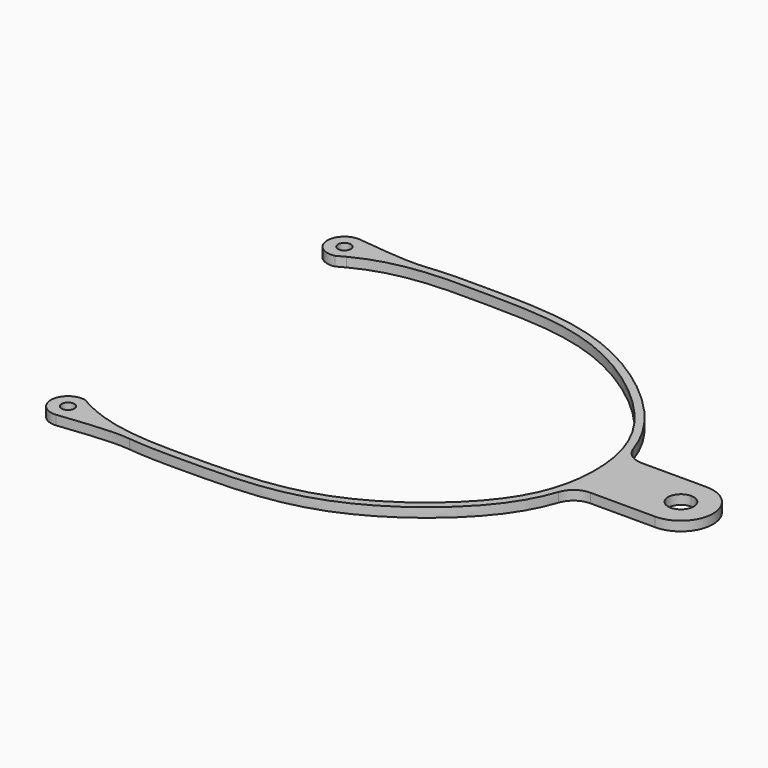
from build123d import *

# Parameters (mm, degrees)
F0_R     = 1.5
F1_DEPTH = 2.2
F2_R     = 5


# Not quite as in the source:
# - ends of sketch curves that miss each other by under 0.0002 mm in the source are joined
# - the dataset's text gives a spline's control points without its knots; the knots are read off the source's solid


with BuildPart() as f1:
    # F0 (on Top) → F1 (new body)
    with BuildSketch(Plane.XY):
        with BuildLine():
            add(Edge.make_bspline(
                [(-30.6111583346, -40.7008057443), (-31.233077321, -40.3790771173), (-31.8528544001, -40.0346551051), (-32.469697118, -39.6698600783)],
                knots=[0.6865550694, 0.6865550694, 0.6865550694, 0.6865550694, 0.698673585, 0.698673585, 0.698673585, 0.698673585], degree=3))
            ThreePointArc((-32.469697118, -39.6698600783), (-37.400344821, -43.2656468064), (-33.0455697059, -47.5407962381))
            add(Edge.make_bspline(
                [(-33.0455697059, -47.5407962381), (-28.2150059427, -47.0976245157), (-21.512714319, -46.0289871022), (-16.6916312134, -46.5655575872)],
                knots=[0, 0, 0, 0, 16.3829910165, 16.3829910165, 16.3829910165, 16.3829910165], degree=3))
            add(Edge.make_bspline(
                [(58.5705779891, -10.6833517733), (58.5045966245, -10.9937274451), (58.1139682264, -12.7078835649), (57.1321161632, -15.8212976201), (55.4627512009, -19.3062888881), (53.7559729129, -22.0784311932), (51.7889797877, -24.8398815578), (48.8824684734, -28.233839645), (44.8027944584, -32.1279022255), (40.2521320917, -35.7428568059), (35.3501612154, -38.9743729453), (31.0709874957, -41.2568133399), (27.5873440069, -42.7817363934), (24.0850094319, -44.0818391055), (19.7200729084, -45.2896051132), (14.5079732054, -46.2040279233), (9.333650913, -46.7087635295), (5.0560116744, -46.8940848045), (1.6559105615, -46.9634870038), (-0.8844247603, -46.9908203291), (-3.4095063019, -47.0107743311), (-5.9465324466, -47.0289364293), (-8.4959599535, -47.0211705077), (-11.9085350935, -46.9496883405), (-14.6448180595, -46.7853276586), (-16.5270909923, -46.5838707043), (-16.6916312134, -46.5655575872)],
                knots=[0.0555924477, 0.0555924477, 0.0555924477, 0.0555924477, 0.0625, 0.09375, 0.125, 0.140625, 0.15625, 0.1875, 0.21875, 0.25, 0.28125, 0.3125, 0.328125, 0.34375, 0.375, 0.40625, 0.4375, 0.46875, 0.484375, 0.5, 0.515625, 0.53125, 0.546875, 0.5625, 0.59375, 0.5967429767, 0.5967429767, 0.5967429767, 0.5967429767], degree=3))
            Line((58.5705779891, -10.6833517733), (77.5044386559, -10.6833535796))
            ThreePointArc((77.5044386559, -10.6833535796), (85.0044386559, -3.1833535796), (77.5044386559, 4.3166464204))
            Line((77.5044386559, 4.3166464204), (58.6926016813, 4.3166464204))
            add(Edge.make_bspline(
                [(59.3254850017, -3.1833535832), (60.0342853265, -2.7966780854), (58.8687853693, -1.6734940692), (59.3856047623, 0.8985285026), (58.9622009071, 3.1879456463), (58.6926016813, 4.3166464204)],
                knots=[0, 0, 0, 0, 0.0130384822, 0.0314878463, 0.049315333, 0.049315333, 0.049315333, 0.049315333], degree=3))
            add(Edge.make_bspline(
                [(57.5012365496, -3.6881837366), (58.3665907715, -3.5375700684), (58.9841699395, -3.3695529499), (59.3254850017, -3.1833535832)],
                knots=[0.9937214612, 0.9937214612, 0.9937214612, 0.9937214612, 1, 1, 1, 1], degree=3))
            add(Edge.make_bspline(
                [(57.5012365496, -3.6881837366), (57.4239325318, -9.7536818174), (53.9530648244, -23.5829729529), (26.6651894068, -45.0062374143), (-2.5492473673, -45.1539383898), (-21.5965397706, -45.3642119383), (-30.6111583346, -40.7008057443)],
                knots=[0.0039126122, 0.0039126122, 0.0039126122, 0.0039126122, 0.1450305925, 0.333052663, 0.5108990784, 0.6865550694, 0.6865550694, 0.6865550694, 0.6865550694], degree=3))
        make_face()
        with Locations((-33.4110080981, -43.5575243692)):
            Circle(F0_R, mode=Mode.SUBTRACT)
        with BuildLine():
            ThreePointArc((77.5044386559, -6.1833535796), (74.5044386559, -3.1833535796), (77.5044386559, -0.1833535796))
            ThreePointArc((77.5044386559, -0.1833535796), (79.6257589995, -1.062033236), (80.5044386559, -3.1833535796))
            ThreePointArc((80.5044386559, -3.1833535796), (79.6257589995, -5.3046739232), (77.5044386559, -6.1833535796))
        make_face(mode=Mode.SUBTRACT)
        with BuildLine():
            ThreePointArc((-35.3506780872, 33.692577605), (-33.9468187682, 33.2268662862), (-32.469697118, 33.3031529191))
            add(Edge.make_bspline(
                [(-30.6111583346, 34.3340985851), (-31.233077321, 34.0123699581), (-31.8528544001, 33.6679479459), (-32.469697118, 33.3031529191)],
                knots=[0.6865550694, 0.6865550694, 0.6865550694, 0.6865550694, 0.698673585, 0.698673585, 0.698673585, 0.698673585], degree=3))
            add(Edge.make_bspline(
                [(57.5044386559, -3.1833535796), (57.5044386559, 3.0581977794), (54.1636559986, 17.0509341089), (26.6651894068, 38.6395302551), (-2.5492473673, 38.7872312306), (-21.5965397706, 38.9975047791), (-30.6111583346, 34.3340985851)],
                knots=[0, 0, 0, 0, 0.1450305925, 0.333052663, 0.5108990784, 0.6865550694, 0.6865550694, 0.6865550694, 0.6865550694], degree=3))
            add(Edge.make_bspline(
                [(57.5044386559, -3.1833535796), (57.5044386559, -3.3517371584), (57.5033798672, -3.5200128066), (57.5012365496, -3.6881837366)],
                knots=[0, 0, 0, 0, 0.0039126122, 0.0039126122, 0.0039126122, 0.0039126122], degree=3))
            add(Edge.make_bspline(
                [(57.5012365496, -3.6881837366), (58.3665907715, -3.5375700684), (58.9841699395, -3.3695529499), (59.3254850017, -3.1833535832)],
                knots=[0.9937214612, 0.9937214612, 0.9937214612, 0.9937214612, 1, 1, 1, 1], degree=3))
            add(Edge.make_bspline(
                [(59.3254850017, -3.1833535832), (60.0342853265, -2.7966780854), (58.8687853693, -1.6734940692), (59.3856047623, 0.8985285026), (58.9622009071, 3.1879456463), (58.6926016813, 4.3166464204)],
                knots=[0, 0, 0, 0, 0.0130384822, 0.0314878463, 0.049315333, 0.049315333, 0.049315333, 0.049315333], degree=3))
            Line((58.6926016813, 4.3166464204), (58.5705864982, 4.3166464204))
            add(Edge.make_bspline(
                [(58.5705864982, 4.3166464204), (58.5045966245, 4.6270202787), (58.1139682264, 6.3411763984), (57.1321161632, 9.4545904537), (55.4627512009, 12.9395817217), (53.7559729129, 15.7117240268), (51.7889797877, 18.4731743913), (48.8824684734, 21.8671324785), (44.8027944584, 25.7611950591), (40.2521320917, 29.3761496394), (35.3501612154, 32.6076657789), (31.0709874957, 34.8901061735), (27.5873440069, 36.4150292269), (24.0850094319, 37.7151319391), (19.7200729084, 38.9228979468), (14.5079732054, 39.8373207569), (9.333650913, 40.3420563631), (5.0560116744, 40.5273776381), (1.6559105615, 40.5967798374), (-0.6449427019, 40.6215364001), (-2.0915209967, 40.6335552581), (-2.6960509898, 40.6382858746)],
                knots=[0.0555924477, 0.0555924477, 0.0555924477, 0.0555924477, 0.0625, 0.09375, 0.125, 0.140625, 0.15625, 0.1875, 0.21875, 0.25, 0.28125, 0.3125, 0.328125, 0.34375, 0.375, 0.40625, 0.4375, 0.46875, 0.484375, 0.5, 0.511206008, 0.511206008, 0.511206008, 0.511206008], degree=3))
            add(Edge.make_bspline(
                [(-2.6960509898, 40.6382858746), (-2.9344421468, 40.6401513521), (-4.0160115872, 40.6484090232), (-5.9465324466, 40.6622292629), (-8.4959599535, 40.6544633413), (-11.9085350935, 40.5829811741), (-14.6448180595, 40.4186204922), (-16.5270909923, 40.2171635379), (-16.6916314281, 40.1988523389)],
                knots=[0.511206008, 0.511206008, 0.511206008, 0.511206008, 0.515625, 0.53125, 0.546875, 0.5625, 0.59375, 0.5967429767, 0.5967429767, 0.5967429767, 0.5967429767], degree=3))
            add(Edge.make_bspline(
                [(-18.3474642287, 40.0770180524), (-17.7760545185, 40.1001547528), (-17.2224405061, 40.1397731224), (-16.6916314281, 40.1988523389)],
                knots=[14.5791963744, 14.5791963744, 14.5791963744, 14.5791963744, 16.3829910165, 16.3829910165, 16.3829910165, 16.3829910165], degree=3))
            add(Edge.make_bspline(
                [(-18.3474642287, 40.0770180524), (-19.3628733695, 39.9392326528), (-22.0032579926, 39.5041891519), (-25.5922390173, 38.5279804037), (-29.0379906327, 37.1641344821), (-31.629223055, 35.9417528172), (-33.6064465264, 34.8002248895), (-34.9272694884, 33.9676196507), (-35.3506780872, 33.692577605)],
                knots=[0.5489272334, 0.5489272334, 0.5489272334, 0.5489272334, 0.5635582322, 0.5867417108, 0.6077658408, 0.6262201744, 0.6449115004, 0.6534319228, 0.6534319228, 0.6534319228, 0.6534319228], degree=3))
        make_face()
        with BuildLine():
            ThreePointArc((-33.0455697059, 41.1740890789), (-37.2336779457, 38.368609737), (-35.3506780872, 33.692577605))
            add(Edge.make_bspline(
                [(-18.3474642287, 40.0770180524), (-19.3628733695, 39.9392326528), (-22.0032579926, 39.5041891519), (-25.5922390173, 38.5279804037), (-29.0379906327, 37.1641344821), (-31.629223055, 35.9417528172), (-33.6064465264, 34.8002248895), (-34.9272694884, 33.9676196507), (-35.3506780872, 33.692577605)],
                knots=[0.5489272334, 0.5489272334, 0.5489272334, 0.5489272334, 0.5635582322, 0.5867417108, 0.6077658408, 0.6262201744, 0.6449115004, 0.6534319228, 0.6534319228, 0.6534319228, 0.6534319228], degree=3))
            add(Edge.make_bspline(
                [(-33.0455697059, 41.1740890789), (-28.7468590717, 40.7797113024), (-22.9658915055, 39.8900153359), (-18.3474642287, 40.0770180524)],
                knots=[0, 0, 0, 0, 14.5791963744, 14.5791963744, 14.5791963744, 14.5791963744], degree=3))
        make_face()
        with Locations((-33.4110080981, 37.19081721)):
            Circle(F0_R, mode=Mode.SUBTRACT)
    extrude(amount=F1_DEPTH)

    # F2
    f2_edges = [f1.edges().sort_by_distance(p)[0] for p in [
        (58.570578, -10.683352, 1.1),
        (58.570586, 4.316646, 1.1),
    ]]
    fillet(f2_edges, radius=F2_R)


solid = f1.part
